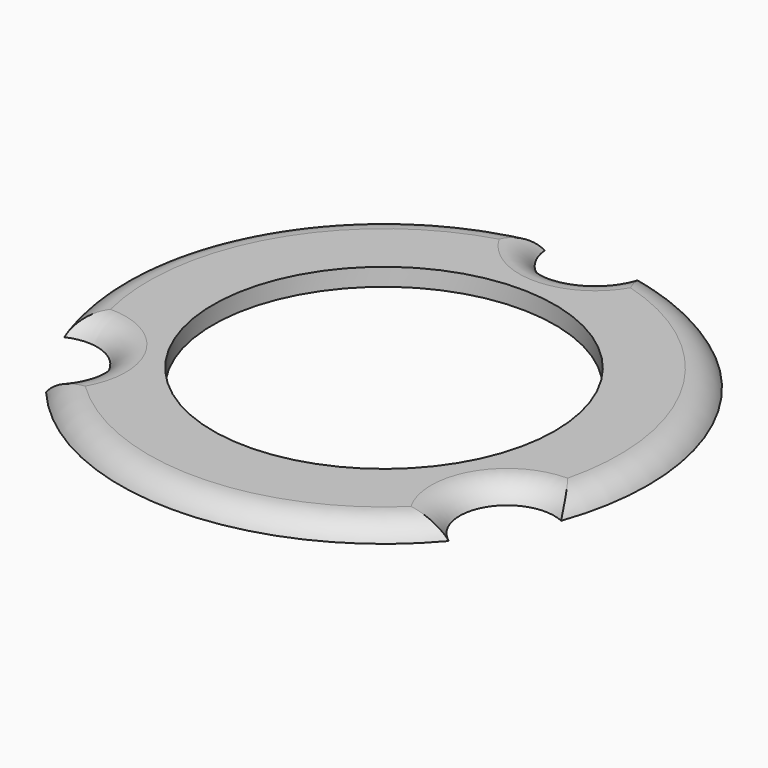
from build123d import *

# Parameters (mm, degrees)
F0_R         = 27.1053686487
F1_DEPTH     = 2.794
F2_T2_ANGLE  = 130.513894387
F2_T4_ANGLE  = 343.3509048615
F2_T6_ANGLE  = 130.513894387
F2_T8_ANGLE  = 343.3509048615
F2_T10_ANGLE = 130.513894387
F2_T12_ANGLE = 343.3509048615


# Not quite as in the source:
# - a fillet or chamfer that OpenCascade refuses, or shapes differently, is made with other operations: its cross-section is extruded or revolved along the edge and cut away or added


with BuildPart() as f1:
    # F0 (on Top) → F1 (new body)
    with BuildSketch(Plane.XY):
        with BuildLine():
            ThreePointArc((39.4058168676, -14.1300394968), (41.2438235607, -7.1710136852), (41.8625897333, 0))
            ThreePointArc((41.8625897333, 0), (32.1326921102, 26.8321918026), (7.4659352731, 41.1914582126))
            ThreePointArc((7.4659352731, 41.1914582126), (0, 34.366550311), (-7.4659352731, 41.1914582126))
            ThreePointArc((-7.4659352731, 41.1914582126), (-36.2540661773, 20.9312948667), (-39.4058168676, -14.1300394968))
            ThreePointArc((-39.4058168676, -14.1300394968), (-32.218910691, -14.6140069025), (-28.758026755, -20.9312948667))
            ThreePointArc((-28.758026755, -20.9312948667), (-29.6008750359, -24.3846489835), (-31.9398815945, -27.0614187158))
            ThreePointArc((-31.9398815945, -27.0614187158), (0, -41.8625897333), (31.9398815945, -27.0614187158))
            ThreePointArc((31.9398815945, -27.0614187158), (29.7623056098, -17.1832751555), (39.4058168676, -14.1300394968))
        make_face()
        Circle(F0_R, mode=Mode.SUBTRACT)
    extrude(amount=F1_DEPTH)

    # F2: fillet of radius 5.08 on 6 edges, made by hand

    # F2_s1 → F2_t2 (revolve, cut)
    with BuildSketch(Plane(origin=(0, 0, 0), x_dir=(0, 0, 1), z_dir=(0.9957938256, -0.0916223607, 0))):
        with BuildLine():
            ThreePointArc((2.794, -37.3260046741), (2.0394641369, -39.9899791484), (0, -41.8625897333))
            Line((0, -41.8625897333), (2.794, -41.8625897333))
            Line((2.794, -41.8625897333), (2.794, -37.3260046741))
        make_face()
    revolve(axis=Axis((0, 0, 2.794), (0, 0, 1)), revolution_arc=F2_T2_ANGLE, mode=Mode.SUBTRACT)

    # F2_s3 → F2_t4 (revolve, cut)
    with BuildSketch(Plane(origin=(3.7584385128, 4.7548188772, 0), x_dir=(0, 0, 1), z_dir=(0.6201152013, 0.7845107629, 0))):
        with BuildLine():
            ThreePointArc((0, 48.9175586674), (2.0394641369, 50.7901692523), (2.794, 53.4541437266))
            Line((2.794, 53.4541437266), (2.794, 48.9175586674))
            Line((2.794, 48.9175586674), (0, 48.9175586674))
        make_face()
    revolve(axis=Axis((36.2540661773, -20.9312948667, 2.794), (0, 0, -1)), revolution_arc=F2_T4_ANGLE, mode=Mode.SUBTRACT)

    # F2_s5 → F2_t6 (revolve, cut)
    with BuildSketch(Plane(origin=(0, 0, 0), x_dir=(0, 0, 1), z_dir=(-0.4185496208, 0.9081939302, 0))):
        with BuildLine():
            ThreePointArc((2.794, -37.3260046741), (2.0394641369, -39.9899791484), (0, -41.8625897333))
            Line((0, -41.8625897333), (2.794, -41.8625897333))
            Line((2.794, -41.8625897333), (2.794, -37.3260046741))
        make_face()
    revolve(axis=Axis((0, 0, 2.794), (0, 0, 1)), revolution_arc=F2_T6_ANGLE, mode=Mode.SUBTRACT)

    # F2_s7 → F2_t8 (revolve, cut)
    with BuildSketch(Plane(origin=(-3.7584385128, 4.7548188772, 0), x_dir=(0, 0, 1), z_dir=(-0.6201152013, 0.7845107629, 0))):
        with BuildLine():
            ThreePointArc((2.794, -53.4541437266), (2.0394641369, -50.7901692523), (0, -48.9175586674))
            Line((0, -48.9175586674), (2.794, -48.9175586674))
            Line((2.794, -48.9175586674), (2.794, -53.4541437266))
        make_face()
    revolve(axis=Axis((-36.2540661773, -20.9312948667, 2.794), (0, 0, 1)), revolution_arc=F2_T8_ANGLE, mode=Mode.SUBTRACT)

    # F2_s9 → F2_t10 (revolve, cut)
    with BuildSketch(Plane(origin=(0, 0, 0), x_dir=(0, 0, 1), z_dir=(-0.9957938256, -0.0916223607, 0))):
        with BuildLine():
            ThreePointArc((2.794, 37.3260046741), (2.0394641369, 39.9899791484), (0, 41.8625897333))
            Line((0, 41.8625897333), (2.794, 41.8625897333))
            Line((2.794, 41.8625897333), (2.794, 37.3260046741))
        make_face()
    revolve(axis=Axis((0, 0, 2.794), (0, 0, -1)), revolution_arc=F2_T10_ANGLE, mode=Mode.SUBTRACT)

    # F2_s11 → F2_t12 (revolve, cut)
    with BuildSketch(Plane(origin=(-5.9970131945, 0.877493792, 0), x_dir=(0, 0, 1), z_dir=(-0.9894638509, 0.1447801361, 0))):
        with BuildLine():
            ThreePointArc((2.794, 53.4541437266), (2.0394641369, 50.7901692523), (0, 48.9175586674))
            Line((0, 48.9175586674), (2.794, 48.9175586674))
            Line((2.794, 48.9175586674), (2.794, 53.4541437266))
        make_face()
    revolve(axis=Axis((0, 41.8625897333, 2.794), (0, 0, -1)), revolution_arc=F2_T12_ANGLE, mode=Mode.SUBTRACT)


solid = f1.part
